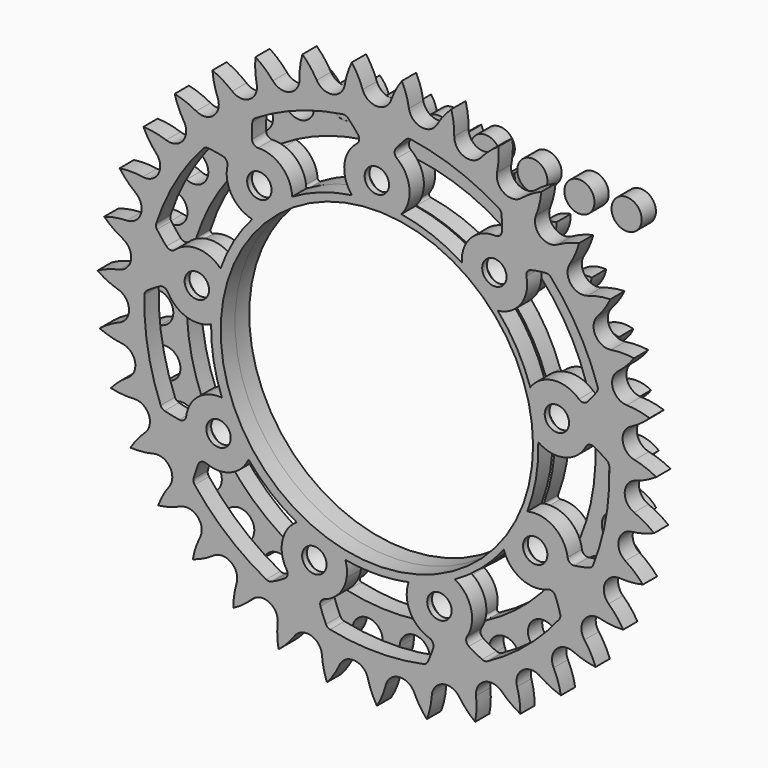
from build123d import *

# Parameters (mm, degrees)
F0_R           = 52.55
F1_DEPTH       = 6
F0_R_2         = 5.07
F2_D           = 8.2
F2_CSINK_D     = 16.2
F2_CSINK_ANGLE = 90
F3_R           = 52.55
F4_DEPTH       = 6
F5_D           = 8.2
F5_CSINK_D     = 16.2
F5_CSINK_ANGLE = 90
F6_D           = 8.2
F6_CSINK_D     = 16.2
F6_CSINK_ANGLE = 90


# Not quite as in the source:
# - a feature names something its author has since deleted; it is built from what else it names


with BuildPart() as f1:
    # F0 (on Front) → F1 (new body)
    with BuildSketch(Plane.XZ):
        with BuildLine():
            ThreePointArc((5.0539361628, 77.9443789243), (0, 73.378314), (-5.0539361628, 77.9443789243))
            ThreePointArc((-5.0539361628, 77.9443789243), (-6.1871728917, 81.776647272), (-8.6369474048, 84.9340371763))
            ThreePointArc((-8.6369474048, 84.9340371763), (-10.4009969746, 81.3481432448), (-10.739606334, 77.3662027789))
            ThreePointArc((-10.739606334, 77.3662027789), (-14.7709460148, 71.8762556016), (-20.6405699194, 75.3315030385))
            ThreePointArc((-20.6405699194, 75.3315030385), (-22.5220391728, 78.8572057516), (-25.5572445727, 81.456827715))
            ThreePointArc((-25.5572445727, 81.456827715), (-26.5633488026, 77.5892366752), (-26.0934680857, 73.6206452016))
            ThreePointArc((-26.0934680857, 73.6206452016), (-28.9371677642, 67.4315748538), (-35.3821763182, 69.6345465672))
            ThreePointArc((-35.3821763182, 69.6345465672), (-37.9348505239, 72.7093409623), (-41.4312251451, 74.6447661563))
            ThreePointArc((-41.4312251451, 74.6447661563), (-41.6381940096, 70.6538176397), (-40.3790601881, 66.8610497596))
            ThreePointArc((-40.3790601881, 66.8610497596), (-41.9186984654, 60.2262375086), (-48.6752322614, 61.0867435777))
            ThreePointArc((-48.6752322614, 61.0867435777), (-51.7946046375, 63.5847472111), (-55.609006492, 64.7767391007))
            ThreePointArc((-55.609006492, 64.7767391007), (-55.0083666616, 60.8258230086), (-53.0115288221, 57.3641550847))
            ThreePointArc((-53.0115288221, 57.3641550847), (-53.1840727262, 50.5552309235), (-59.9755184767, 50.0380421288))
            ThreePointArc((-59.9755184767, 50.0380421288), (-63.5338815515, 51.8569864381), (-67.5101485793, 52.2567447354))
            ThreePointArc((-67.5101485793, 52.2567447354), (-66.1264903192, 48.5076120368), (-63.4736992375, 45.5187651606))
            ThreePointArc((-63.4736992375, 45.5187651606), (-62.2720848007, 38.8144872445), (-68.8203999187, 36.9407773559))
            ThreePointArc((-68.8203999187, 36.9407773559), (-72.67207389, 38.0061945474), (-76.6474172517, 37.5973531007))
            ThreePointArc((-76.6474172517, 37.5973531007), (-74.5373876936, 34.2034937288), (-71.3372489483, 31.8098316426))
            ThreePointArc((-71.3372489483, 31.8098316426), (-68.8106704069, 25.4846738971), (-74.847766102, 22.3311528177))
            ThreePointArc((-74.847766102, 22.3311528177), (-78.8350629847, 22.5994245865), (-82.6467316562, 21.3987214126))
            ThreePointArc((-82.6467316562, 21.3987214126), (-79.8967156581, 18.4990803688), (-76.2802433053, 16.7985998796))
            ThreePointArc((-76.2802433053, 16.7985998796), (-72.5321390816, 11.1115150061), (-77.8108559469, 6.8072882593))
            ThreePointArc((-77.8108559469, 6.8072882593), (-81.7705353382, 6.2674315276), (-85.262479156, 4.3240235556))
            ThreePointArc((-85.262479156, 4.3240235556), (-81.9850626961, 2.0373124849), (-78.1003155389, 1.0996314638))
            ThreePointArc((-78.1003155389, 1.0996314638), (-73.2841334602, -3.7165506149), (-77.5883602069, -8.9952674802))
            ThreePointArc((-77.5883602069, -8.9952674802), (-81.3583123673, -10.3211509144), (-84.3875707413, -12.9277003338))
            ThreePointArc((-84.3875707413, -12.9277003338), (-80.7169316345, -14.5078632114), (-76.7229516779, -14.6443559933))
            ThreePointArc((-76.7229516779, -14.6443559933), (-71.0358668044, -18.392460217), (-74.1893878838, -24.4295559122))
            ThreePointArc((-74.1893878838, -24.4295559122), (-77.6152705288, -26.4871842253), (-80.0578252653, -29.6501626526))
            ThreePointArc((-80.0578252653, -29.6501626526), (-76.1442399079, -30.4590852833), (-72.2045411607, -29.7888017954))
            ThreePointArc((-72.2045411607, -29.7888017954), (-65.8793834152, -32.3153803368), (-67.7530933038, -38.8636954547))
            ThreePointArc((-67.7530933038, -38.8636954547), (-70.6946503955, -41.5688291019), (-72.4505030166, -45.1587438287))
            ThreePointArc((-72.4505030166, -45.1587438287), (-68.4541940529, -45.1633088249), (-64.7300682447, -43.7136905519))
            ThreePointArc((-64.7300682447, -43.7136905519), (-58.0257903286, -44.9153049887), (-58.5429791233, -51.7067507391))
            ThreePointArc((-58.5429791233, -51.7067507391), (-60.8797829688, -54.9486412309), (-61.8770486618, -58.8185207264))
            ThreePointArc((-61.8770486618, -58.8185207264), (-57.9616254504, -58.0185411967), (-54.6055387293, -55.8489356812))
            ThreePointArc((-54.6055387293, -55.8489356812), (-47.7966145682, -55.676391777), (-46.936108499, -62.432925573))
            ThreePointArc((-46.936108499, -62.432925573), (-48.5724900742, -66.0788495317), (-48.7703406645, -70.0702604748))
            ThreePointArc((-48.7703406645, -70.0702604748), (-45.0961010917, -68.4984876751), (-42.2454520424, -65.6977188216))
            ThreePointArc((-42.2454520424, -65.6977188216), (-35.6106397914, -64.1580805443), (-33.407668078, -70.6030890983))
            ThreePointArc((-33.407668078, -70.6030890983), (-34.276633729, -74.5037819688), (-33.6669691902, -78.4533155264))
            ThreePointArc((-33.6669691902, -78.4533155264), (-30.3843370557, -76.1740980198), (-28.1558315853, -72.8568296344))
            ThreePointArc((-28.1558315853, -72.8568296344), (-21.9667612376, -70.0131299558), (-18.5115138007, -75.8827538604))
            ThreePointArc((-18.5115138007, -75.8827538604), (-18.5774879716, -79.8785208183), (-17.1852680415, -83.6244826225))
            ThreePointArc((-17.1852680415, -83.6244826225), (-14.4286346907, -80.7311318415), (-12.9135080749, -77.0331732816))
            ThreePointArc((-12.9135080749, -77.0331732816), (-7.4235608976, -73.0018336008), (-2.8574959733, -78.0557697636))
            ThreePointArc((-2.8574959733, -78.0557697636), (-2.1177776738, -81.9830236401), (0, -85.3720535746))
            ThreePointArc((0, -85.3720535746), (2.1177776738, -81.9830236401), (2.8574959733, -78.0557697636))
            ThreePointArc((2.8574959733, -78.0557697636), (7.4235608976, -73.0018336008), (12.9135080749, -77.0331732816))
            ThreePointArc((12.9135080749, -77.0331732816), (14.4286346907, -80.7311318415), (17.1852680415, -83.6244826225))
            ThreePointArc((17.1852680415, -83.6244826225), (18.5774879716, -79.8785208183), (18.5115138007, -75.8827538604))
            ThreePointArc((18.5115138007, -75.8827538604), (21.9667612376, -70.0131299558), (28.1558315853, -72.8568296344))
            ThreePointArc((28.1558315853, -72.8568296344), (30.3843370557, -76.1740980198), (33.6669691902, -78.4533155264))
            ThreePointArc((33.6669691902, -78.4533155264), (34.276633729, -74.5037819688), (33.407668078, -70.6030890983))
            ThreePointArc((33.407668078, -70.6030890983), (35.6106397914, -64.1580805443), (42.2454520424, -65.6977188216))
            ThreePointArc((42.2454520424, -65.6977188216), (45.0961010917, -68.4984876751), (48.7703406645, -70.0702604748))
            ThreePointArc((48.7703406645, -70.0702604748), (48.5724900742, -66.0788495317), (46.936108499, -62.432925573))
            ThreePointArc((46.936108499, -62.432925573), (47.7966145682, -55.676391777), (54.6055387293, -55.8489356812))
            ThreePointArc((54.6055387293, -55.8489356812), (57.9616254504, -58.0185411967), (61.8770486618, -58.8185207264))
            ThreePointArc((61.8770486618, -58.8185207264), (60.8797829688, -54.9486412309), (58.5429791233, -51.7067507391))
            ThreePointArc((58.5429791233, -51.7067507391), (58.0257903286, -44.9153049887), (64.7300682447, -43.7136905519))
            ThreePointArc((64.7300682447, -43.7136905519), (68.4541940529, -45.1633088249), (72.4505030166, -45.1587438287))
            ThreePointArc((72.4505030166, -45.1587438287), (70.6946503955, -41.5688291019), (67.7530933038, -38.8636954547))
            ThreePointArc((67.7530933038, -38.8636954547), (65.8793834152, -32.3153803368), (72.2045411607, -29.7888017954))
            ThreePointArc((72.2045411607, -29.7888017954), (76.1442399079, -30.4590852833), (80.0578252653, -29.6501626526))
            ThreePointArc((80.0578252653, -29.6501626526), (77.6152705288, -26.4871842253), (74.1893878838, -24.4295559122))
            ThreePointArc((74.1893878838, -24.4295559122), (71.0358668044, -18.392460217), (76.7229516779, -14.6443559933))
            ThreePointArc((76.7229516779, -14.6443559933), (80.7169316345, -14.5078632114), (84.3875707413, -12.9277003338))
            ThreePointArc((84.3875707413, -12.9277003338), (81.3583123673, -10.3211509144), (77.5883602069, -8.9952674802))
            ThreePointArc((77.5883602069, -8.9952674802), (73.2841334602, -3.7165506149), (78.1003155389, 1.0996314638))
            ThreePointArc((78.1003155389, 1.0996314638), (81.9850626961, 2.0373124849), (85.262479156, 4.3240235556))
            ThreePointArc((85.262479156, 4.3240235556), (81.7705353382, 6.2674315276), (77.8108559469, 6.8072882593))
            ThreePointArc((77.8108559469, 6.8072882593), (72.5321390816, 11.1115150061), (76.2802433053, 16.7985998796))
            ThreePointArc((76.2802433053, 16.7985998796), (79.8967156581, 18.4990803688), (82.6467316562, 21.3987214126))
            ThreePointArc((82.6467316562, 21.3987214126), (78.8350629847, 22.5994245865), (74.847766102, 22.3311528177))
            ThreePointArc((74.847766102, 22.3311528177), (68.8106704069, 25.4846738971), (71.3372489483, 31.8098316426))
            ThreePointArc((71.3372489483, 31.8098316426), (74.5373876936, 34.2034937288), (76.6474172517, 37.5973531007))
            ThreePointArc((76.6474172517, 37.5973531007), (72.67207389, 38.0061945474), (68.8203999187, 36.9407773559))
            ThreePointArc((68.8203999187, 36.9407773559), (62.2720848007, 38.8144872445), (63.4736992375, 45.5187651606))
            ThreePointArc((63.4736992375, 45.5187651606), (66.1264903192, 48.5076120368), (67.5101485793, 52.2567447354))
            ThreePointArc((67.5101485793, 52.2567447354), (63.5338815515, 51.8569864381), (59.9755184767, 50.0380421288))
            ThreePointArc((59.9755184767, 50.0380421288), (53.1840727262, 50.5552309235), (53.0115288221, 57.3641550847))
            ThreePointArc((53.0115288221, 57.3641550847), (55.0083666616, 60.8258230086), (55.609006492, 64.7767391007))
            ThreePointArc((55.609006492, 64.7767391007), (51.7946046375, 63.5847472111), (48.6752322614, 61.0867435777))
            ThreePointArc((48.6752322614, 61.0867435777), (41.9186984654, 60.2262375086), (40.3790601881, 66.8610497596))
            ThreePointArc((40.3790601881, 66.8610497596), (41.6381940096, 70.6538176397), (41.4312251451, 74.6447661563))
            ThreePointArc((41.4312251451, 74.6447661563), (37.9348505239, 72.7093409623), (35.3821763182, 69.6345465672))
            ThreePointArc((35.3821763182, 69.6345465672), (28.9371677642, 67.4315748538), (26.0934680857, 73.6206452016))
            ThreePointArc((26.0934680857, 73.6206452016), (26.5633488026, 77.5892366752), (25.5572445727, 81.456827715))
            ThreePointArc((25.5572445727, 81.456827715), (22.5220391728, 78.8572057516), (20.6405699194, 75.3315030385))
            ThreePointArc((20.6405699194, 75.3315030385), (14.7709460148, 71.8762556016), (10.739606334, 77.3662027789))
            ThreePointArc((10.739606334, 77.3662027789), (10.4009969746, 81.3481432448), (8.6369474048, 84.9340371763))
            ThreePointArc((8.6369474048, 84.9340371763), (6.1871728917, 81.776647272), (5.0539361628, 77.9443789243))
        make_face()
        with BuildLine():
            ThreePointArc((-54.4759158417, -41.93959675), (-54.5447016016, -41.1315886082), (-53.8383054337, -40.7333260165))
            ThreePointArc((-53.8383054337, -40.7333260165), (-48.0309187527, -39.2735438367), (-44.0987264454, -34.7575093225))
            ThreePointArc((-44.0987264454, -34.7575093225), (-43.5114164609, -34.3147443915), (-42.8280957261, -34.5868593957))
            ThreePointArc((-42.8280957261, -34.5868593957), (-35.3854239296, -42.1707055316), (-26.6243883257, -48.1833871988))
            ThreePointArc((-26.6243883257, -48.1833871988), (-26.2377500975, -48.8090744024), (-26.5718029893, -49.4643470644))
            ThreePointArc((-26.5718029893, -49.4643470644), (-30.3364098723, -54.1210028385), (-30.7655709797, -60.093651223))
            ThreePointArc((-30.7655709797, -60.093651223), (-31.0351185634, -60.8584733913), (-31.8427958991, -60.9310417763))
            ThreePointArc((-31.8427958991, -60.9310417763), (-44.1916130719, -52.665515334), (-54.4759158417, -41.93959675))
        make_face(mode=Mode.SUBTRACT)
        with BuildLine():
            ThreePointArc((-68.6892257605, 2.8888486924), (-68.2225410875, 3.5520334735), (-67.4254119691, 3.4030576147))
            ThreePointArc((-67.4254119691, 3.4030576147), (-62.0383657751, 0.7883994384), (-56.1232806782, 1.7203180889))
            ThreePointArc((-56.1232806782, 1.7203180889), (-55.3887713165, 1.6819801228), (-55.0402294178, 1.0342978342))
            ThreePointArc((-55.0402294178, 1.0342978342), (-54.2136143761, -9.5593225694), (-51.3671490125, -19.7967890831))
            ThreePointArc((-51.3671490125, -19.7967890831), (-51.4731509283, -20.524619551), (-52.1502514379, -20.8118624726))
            ThreePointArc((-52.1502514379, -20.8118624726), (-58.0273482552, -21.9592250922), (-62.1952491153, -26.2586797555))
            ThreePointArc((-62.1952491153, -26.2586797555), (-62.8933527575, -26.6713056804), (-63.558715551, -26.2077313044))
            ThreePointArc((-63.558715551, -26.2077313044), (-67.7054803406, -11.938304031), (-68.6892257605, 2.8888486924))
        make_face(mode=Mode.SUBTRACT)
        with BuildLine():
            ThreePointArc((10.5762195558, -54.0244429456), (11.274585604, -54.2552208885), (11.4398873906, -54.9719139298))
            ThreePointArc((11.4398873906, -54.9719139298), (11.5492718416, -60.9589618687), (15.0596597386, -65.8101354168))
            ThreePointArc((15.0596597386, -65.8101354168), (15.3447925233, -66.5692850359), (14.7727218472, -67.1440406279))
            ThreePointArc((14.7727218472, -67.1440406279), (1.0883e-06, -68.7499467003), (-14.7727194682, -67.1440387664))
            ThreePointArc((-14.7727194682, -67.1440387664), (-15.3447900394, -66.5692832535), (-15.0596574397, -65.810133704))
            ThreePointArc((-15.0596574397, -65.810133704), (-11.5492710417, -60.9589594738), (-11.4398880061, -54.9719118352))
            ThreePointArc((-11.4398880061, -54.9719118352), (-11.2745862677, -54.2552186391), (-10.5762200628, -54.0244407242))
            ThreePointArc((-10.5762200628, -54.0244407242), (-3.612e-07, -55.0499467003), (10.5762195558, -54.0244429456))
        make_face(mode=Mode.SUBTRACT)
        with BuildLine():
            ThreePointArc((31.842796525, -60.9310388211), (31.0351193206, -60.8584704293), (30.7655716397, -60.0936484332))
            ThreePointArc((30.7655716397, -60.0936484332), (30.3364089456, -54.1210004897), (26.5718011715, -49.4643458555))
            ThreePointArc((26.5718011715, -49.4643458555), (26.2377481432, -48.8090731059), (26.6243865094, -48.183385823))
            ThreePointArc((26.6243865094, -48.183385823), (35.3854233761, -42.1707059959), (42.8280967655, -34.5868614233))
            ThreePointArc((42.8280967655, -34.5868614233), (43.5114173983, -34.3147465412), (44.0987273203, -34.7575113226))
            ThreePointArc((44.0987273203, -34.7575113226), (48.0309209049, -39.2735451572), (53.8383082957, -40.7333258508))
            ThreePointArc((53.8383082957, -40.7333258508), (54.5447046501, -41.1315883769), (54.4759188607, -41.9395966468))
            ThreePointArc((54.4759188607, -41.9395966468), (44.1916147393, -52.6655139349), (31.842796525, -60.9310388211))
        make_face(mode=Mode.SUBTRACT)
        with BuildLine():
            ThreePointArc((63.5587141308, -26.2077286383), (62.8933514335, -26.6713029247), (62.1952478277, -26.2586771941))
            ThreePointArc((62.1952478277, -26.2586771941), (58.0273460356, -21.9592238886), (52.1502492683, -20.8118627151))
            ThreePointArc((52.1502492683, -20.8118627151), (51.4731485978, -20.524619814), (51.3671467368, -19.7967891966))
            ThreePointArc((51.3671467368, -19.7967891966), (54.2136142506, -9.5593232809), (55.0402315174, 1.0342969491))
            ThreePointArc((55.0402315174, 1.0342969491), (55.3887734164, 1.6819790786), (56.1232826341, 1.7203171191))
            ThreePointArc((56.1232826341, 1.7203171191), (62.0383682726, 0.7883998102), (67.4254140551, 3.4030595812))
            ThreePointArc((67.4254140551, 3.4030595812), (68.2225432742, 3.5520356103), (68.6892280069, 2.888850712))
            ThreePointArc((68.6892280069, 2.888850712), (67.7054807186, -11.9383018874), (63.5587141308, -26.2077286383))
        make_face(mode=Mode.SUBTRACT)
        with BuildLine():
            ThreePointArc((-50.7620835502, 46.3655697256), (-49.9782953896, 46.5736196166), (-49.4634188942, 45.9471127671))
            ThreePointArc((-49.4634188942, 45.9471127671), (-47.0173719717, 40.4814418542), (-41.8871281409, 37.3931895473))
            ThreePointArc((-41.8871281409, 37.3931895473), (-41.3491044955, 36.8916874445), (-41.498428061, 36.1714956125))
            ThreePointArc((-41.498428061, 36.1714956125), (-47.6746521388, 27.524973663), (-52.074649794, 17.8529466615))
            ThreePointArc((-52.074649794, 17.8529466615), (-52.6236923793, 17.3635328941), (-53.3270176532, 17.5787238682))
            ThreePointArc((-53.3270176532, 17.5787238682), (-58.5666454874, 20.4775181244), (-64.5230789667, 19.8630198024))
            ThreePointArc((-64.5230789667, 19.8630198024), (-65.3230882145, 19.9956623769), (-65.5348058201, 20.7784679112))
            ThreePointArc((-65.5348058201, 20.7784679112), (-59.5392008954, 34.3749724076), (-50.7620835502, 46.3655697256))
        make_face(mode=Mode.SUBTRACT)
        with BuildLine():
            ThreePointArc((-9.0827982891, 68.1473253883), (-8.348649832, 67.8028915329), (-8.356942394, 66.9920032105))
            ThreePointArc((-8.356942394, 66.9920032105), (-9.9964272829, 61.2327677253), (-8.0515228228, 55.5693720375))
            ThreePointArc((-8.0515228228, 55.5693720375), (-7.9617321369, 54.8393642055), (-8.5390510107, 54.3836485923))
            ThreePointArc((-8.5390510107, 54.3836485923), (-18.8281903211, 51.7300288125), (-28.4158431917, 47.1490902497))
            ThreePointArc((-28.4158431917, 47.1490902497), (-29.1510233189, 47.1270953238), (-29.5514796447, 47.7440299453))
            ThreePointArc((-29.5514796447, 47.7440299453), (-31.7019584003, 53.3326030283), (-36.6598430755, 56.6905916418))
            ThreePointArc((-36.6598430755, 56.6905916418), (-37.1874247107, 57.3064377811), (-36.8464321078, 58.0421910643))
            ThreePointArc((-36.8464321078, 58.0421910643), (-23.5138676467, 64.6038172215), (-9.0827982891, 68.1473253883))
        make_face(mode=Mode.SUBTRACT)
        with Locations((5.4201e-06, 5.32997e-05)):
            Circle(F0_R, mode=Mode.SUBTRACT)
        with BuildLine():
            ThreePointArc((65.5348030184, 20.7784690407), (65.3230854289, 19.9956636369), (64.523076334, 19.8630209369))
            ThreePointArc((64.523076334, 19.8630209369), (58.5666430134, 20.4775176196), (53.327016147, 17.5787222879))
            ThreePointArc((53.327016147, 17.5787222879), (52.6236907632, 17.3635311946), (52.0746481238, 17.8529451117))
            ThreePointArc((52.0746481238, 17.8529451117), (47.6746525, 27.5249730373), (41.4984302383, 36.1714962841))
            ThreePointArc((41.4984302383, 36.1714962841), (41.3491067754, 36.8916879944), (41.8871302625, 37.3931900616))
            ThreePointArc((41.8871302625, 37.3931900616), (47.0173736459, 40.4814437444), (49.4634192281, 45.9471156144))
            ThreePointArc((49.4634192281, 45.9471156144), (49.9782956912, 46.5736226589), (50.7620839729, 46.3655727167))
            ThreePointArc((50.7620839729, 46.3655727167), (59.5391998071, 34.3749742927), (65.5348030184, 20.7784690407))
        make_face(mode=Mode.SUBTRACT)
        with BuildLine():
            ThreePointArc((36.8464292355, 58.0421901287), (37.1874217669, 57.3064369558), (36.6598403294, 56.6905908186))
            ThreePointArc((36.6598403294, 56.6905908186), (31.7019568296, 53.3326010513), (29.5514795067, 47.7440277666))
            ThreePointArc((29.5514795067, 47.7440277666), (29.1510231733, 47.1270929831), (28.4158429084, 47.1490879889))
            ThreePointArc((28.4158429084, 47.1490879889), (18.8281909999, 51.7300285654), (8.539052247, 54.3836505063))
            ThreePointArc((8.539052247, 54.3836505063), (7.96173353, 54.8393660922), (8.0515241176, 55.5693737953))
            ThreePointArc((8.0515241176, 55.5693737953), (9.9964273504, 61.2327702494), (8.3569408196, 66.9920056063))
            ThreePointArc((8.3569408196, 66.9920056063), (8.3486481074, 67.8028940573), (9.0827966903, 68.1473279513))
            ThreePointArc((9.0827966903, 68.1473279513), (23.5138656014, 64.6038179659), (36.8464292355, 58.0421901287))
        make_face(mode=Mode.SUBTRACT)
    extrude(amount=-F1_DEPTH)

    # F2 (through all)
    with Locations(Plane.XZ):
        with Locations((-60.5657293002, 10.6793721819), (-39.5314722561, 47.1117740818), (0, 61.5000532997), (39.5314722561, 47.1117740818), (60.5657293002, 10.6793721819), (53.2606084916, -30.7500266499), (21.0342570441, -57.7911462637), (-21.0342570441, -57.7911462637), (-53.2606084916, -30.7500266499)):
            CounterSinkHole(F2_D / 2, F2_CSINK_D / 2, counter_sink_angle=F2_CSINK_ANGLE)


with BuildPart() as f1b:
    # F0 (on Front) → F1, piece 2 (new body)
    with BuildSketch(Plane.XZ):
        with Locations((-15.7935424969, 76.8522677032)):
            Circle(F0_R_2)
    extrude(amount=-F1_DEPTH)


with BuildPart() as f1c:
    # F0 (on Front) → F1, piece 3 (new body)
    with BuildSketch(Plane.XZ):
        with Locations((0, 78.458314)):
            Circle(F0_R_2)
    extrude(amount=-F1_DEPTH)


with BuildPart() as f1d:
    # F0 (on Front) → F1, piece 4 (new body)
    with BuildSketch(Plane.XZ):
        with Locations((15.8799886703, 78.458314)):
            Circle(F0_R_2)
    extrude(amount=-F1_DEPTH)


with BuildPart() as f1e:
    # F0 (on Front) → F1, piece 5 (new body)
    with BuildSketch(Plane.XZ):
        with Locations((31.7430435847, 77.8425918352)):
            Circle(F0_R_2)
    extrude(amount=-F1_DEPTH)


with BuildPart() as f1f:
    # F0 (on Front) → F1, piece 6 (new body)
    with BuildSketch(Plane.XZ):
        with Locations((47.5038162957, 75.9416266721)):
            Circle(F0_R_2)
    extrude(amount=-F1_DEPTH)


with BuildPart() as f1g:
    # F0 (on Front) → F1, piece 7 (new body)
    with BuildSketch(Plane.XZ):
        with Locations((63.3414363061, 74.8528579142)):
            Circle(F0_R_2)
    extrude(amount=-F1_DEPTH)


with BuildPart() as f1h:
    # F0 (on Front) → F1, piece 8 (new body)
    with BuildSketch(Plane.XZ):
        with Locations((79.2164363061, 74.8528579142)):
            Circle(F0_R_2)
    extrude(amount=-F1_DEPTH)


with BuildPart() as f4:
    # F3 (on Front) → F4 (new body)
    with BuildSketch(Plane.XZ):
        with BuildLine():
            ThreePointArc((4.7900344729, 86.8582642793), (2.88e-07, 83.47), (-4.7900342811, 86.8582637362))
            ThreePointArc((-4.7900342811, 86.8582637362), (-6.3574974769, 90.4284112682), (-8.4356319096, 93.7275401761))
            ThreePointArc((-8.4356319096, 93.7275401761), (-9.8912869388, 90.1103646743), (-10.796085309, 86.3177099202))
            ThreePointArc((-10.796085309, 86.3177099202), (-14.9041437255, 82.1286028118), (-20.2221983199, 84.6071220571))
            ThreePointArc((-20.2221983199, 84.6071220571), (-22.4019461946, 87.8400144886), (-25.0357663654, 90.7150598063))
            ThreePointArc((-25.0357663654, 90.7150598063), (-25.8221567938, 86.8960965611), (-26.0352100261, 83.0028333418))
            ThreePointArc((-26.0352100261, 83.0028333418), (-29.3292562964, 78.1475247535), (-35.0044042658, 79.6366378602))
            ThreePointArc((-35.0044042658, 79.6366378602), (-37.7263779292, 82.4283673683), (-40.8312306906, 84.7869227739))
            ThreePointArc((-40.8312306906, 84.7869227739), (-40.9230812829, 80.8889164061), (-40.437541671, 77.0201774048))
            ThreePointArc((-40.437541671, 77.0201774048), (-42.8117024378, 71.6547209497), (-48.6615398569, 72.1065665972))
            ThreePointArc((-48.6615398569, 72.1065665972), (-51.8382528358, 74.3674046985), (-55.3143456654, 76.1336642805))
            ThreePointArc((-55.3143456654, 76.1336642805), (-54.708704268, 72.2818999222), (-53.5401774546, 68.5620295937))
            ThreePointArc((-53.5401774546, 68.5620295937), (-54.9181452373, 62.8588754568), (-60.7546535182, 62.2589309543))
            ThreePointArc((-60.7546535182, 62.2589309543), (-64.2840036436, 63.916212452), (-68.0196120578, 65.0334071742))
            ThreePointArc((-68.0196120578, 65.0334071742), (-66.7359444834, 61.351683701), (-64.9219878817, 57.9002417383))
            ThreePointArc((-64.9219878817, 57.9002417383), (-65.259473662, 52.0426939863), (-70.8950626263, 50.4102420436))
            ThreePointArc((-70.8950626263, 50.4102420436), (-74.6636136813, 51.4107005468), (-78.5386721518, 51.8429228516))
            ThreePointArc((-78.5386721518, 51.8429228516), (-76.6182365326, 48.4495738853), (-74.2171522003, 45.377492473))
            ThreePointArc((-74.2171522003, 45.377492473), (-73.5033089076, 39.5538175102), (-78.7568460889, 36.9413264761))
            ThreePointArc((-78.7568460889, 36.9413264761), (-82.6434737418, 37.2528064253), (-86.5334347011, 36.9861643321))
            ThreePointArc((-86.5334347011, 36.9861643321), (-84.037955418, 33.9902549005), (-81.1269161812, 31.3962732629))
            ThreePointArc((-81.1269161812, 31.3962732629), (-79.3846873262, 25.7936487944), (-84.0873197169, 22.2850862801))
            ThreePointArc((-84.0873197169, 22.2850862801), (-87.9671045569, 21.8975764534), (-91.7469414591, 20.9406400586))
            ThreePointArc((-91.7469414591, 20.9406400586), (-88.7566252695, 18.438461156), (-85.4291943245, 16.4059519972))
            ThreePointArc((-85.4291943245, 16.4059519972), (-82.7145765761, 11.2044509832), (-86.7151577019, 6.9125850749))
            ThreePointArc((-86.7151577019, 6.9125850749), (-90.4634002521, 5.838540357), (-94.011626029, 4.2220663837))
            ThreePointArc((-94.011626029, 4.2220663837), (-90.6225841557, 2.2940400987), (-86.9857078709, 0.8883299355))
            ThreePointArc((-86.9857078709, 0.8883299355), (-83.3859512771, -3.7448671016), (-86.5558991689, -8.6820923023))
            ThreePointArc((-86.5558991689, -8.6820923023), (-90.0521278295, -10.4081512304), (-93.2546995853, -12.6322079788))
            ThreePointArc((-93.2546995853, -12.6322079788), (-89.5758586227, -13.924113295), (-85.7464291942, -14.6578437813))
            ThreePointArc((-85.7464291942, -14.6578437813), (-81.3772328939, -18.5738220766), (-83.6146628182, -23.9977200893))
            ThreePointArc((-83.6146628182, -23.9977200893), (-86.7465059235, -26.3203162735), (-89.5004903667, -29.080472783))
            ThreePointArc((-89.5004903667, -29.080472783), (-85.6500912902, -29.6947342305), (-81.7511897308, -29.7329023385))
            ThreePointArc((-81.7511897308, -29.7329023385), (-76.7529832881, -32.8057991273), (-77.9859824061, -38.5420414072))
            ThreePointArc((-77.9859824061, -38.5420414072), (-80.6527799417, -41.3865246951), (-82.8696617465, -44.5940672645))
            ThreePointArc((-82.8696617465, -44.5940672645), (-78.9714595505, -44.510941975), (-75.1283997643, -43.8523209502))
            ThreePointArc((-75.1283997643, -43.8523209502), (-69.6618296468, -45.9833708014), (-69.8507683524, -51.8475898018))
            ThreePointArc((-69.8507683524, -51.8475898018), (-71.9668072513, -55.12253616), (-73.5753340124, -58.6743717319))
            ThreePointArc((-73.5753340124, -58.6743717319), (-69.754620123, -57.8965314206), (-66.0909212136, -56.5622898847))
            ThreePointArc((-66.0909212136, -56.5622898847), (-60.3316874827, -57.6829991028), (-59.4704931305, -63.4867139998))
            ThreePointArc((-59.4704931305, -63.4867139998), (-60.9677621614, -67.0868639578), (-61.9162345051, -70.8688336145))
            ThreePointArc((-61.9162345051, -70.8688336145), (-58.2958098104, -69.421278709), (-54.9292260753, -67.4543002828))
            ThreePointArc((-54.9292260753, -67.4543002828), (-49.0624352419, -67.5286483512), (-47.1787873269, -73.0853229729))
            ThreePointArc((-47.1787873269, -73.0853229729), (-48.0091630312, -76.8949647488), (-48.267096276, -80.7855128736))
            ThreePointArc((-48.267096276, -80.7855128736), (-44.9633242045, -78.7147689796), (-42.002060415, -76.1782739681))
            ThreePointArc((-42.002060415, -76.1782739681), (-36.2162759636, -75.2038712789), (-33.3707164797, -80.3349095307))
            ThreePointArc((-33.3707164797, -80.3349095307), (-33.507509899, -84.2315981033), (-33.0666138582, -88.1056792785))
            ThreePointArc((-33.0666138582, -88.1056792785), (-30.1856803628, -85.4783018086), (-27.7249139736, -82.4538152485))
            ThreePointArc((-27.7249139736, -82.4538152485), (-22.2060957771, -80.4619799057), (-18.4900833474, -85.0024659965))
            ThreePointArc((-18.4900833474, -85.0024659965), (-17.9288978287, -88.8609585888), (-16.8033432638, -92.5940566577))
            ThreePointArc((-16.8033432638, -92.5940566577), (-14.4378439173, -89.4944916856), (-12.5566659849, -86.0792230635))
            ThreePointArc((-12.5566659849, -86.0792230635), (-7.482193401, -83.133974294), (-3.0151637226, -86.9379732649))
            ThreePointArc((-3.0151637226, -86.9379732649), (-1.7740362302, -90.6342547502), (6.09e-07, -94.1063848693))
            ThreePointArc((6.09e-07, -94.1063848693), (1.7740367111, -90.6342549635), (3.0151635802, -86.937973823))
            ThreePointArc((3.0151635802, -86.937973823), (7.4821928273, -83.1339743456), (12.5566657452, -86.0792225397))
            ThreePointArc((12.5566657452, -86.0792225397), (14.4378443525, -89.4944913898), (16.8033444622, -92.5940564402))
            ThreePointArc((16.8033444622, -92.5940564402), (17.92889834, -88.8609587128), (18.490083307, -85.0024665711))
            ThreePointArc((18.490083307, -85.0024665711), (22.2060952218, -80.4619800589), (27.7249136442, -82.4538147759))
            ThreePointArc((27.7249136442, -82.4538147759), (30.1856807381, -85.4783014398), (33.0666149985, -88.1056788505))
            ThreePointArc((33.0666149985, -88.1056788505), (33.5075104243, -84.231598134), (33.3707165425, -80.3349101033))
            ThreePointArc((33.3707165425, -80.3349101033), (36.2162754447, -75.2038715288), (42.0020600065, -76.178273562))
            ThreePointArc((42.0020600065, -76.178273562), (44.963324508, -78.7147685498), (48.2670973215, -80.7855122489))
            ThreePointArc((48.2670973215, -80.7855122489), (48.0091635535, -76.8949646852), (47.1787874909, -73.085323525))
            ThreePointArc((47.1787874909, -73.085323525), (49.0624347759, -67.5286486898), (54.9292256009, -67.4542999561))
            ThreePointArc((54.9292256009, -67.4542999561), (58.2958100322, -69.4212782319), (61.9162354223, -70.8688328131))
            ThreePointArc((61.9162354223, -70.8688328131), (60.967762664, -67.086863802), (59.4704933905, -63.4867145138))
            ThreePointArc((59.4704933905, -63.4867145138), (60.3316870846, -57.6829995191), (66.0909206885, -56.562289648))
            ThreePointArc((66.0909206885, -56.562289648), (69.7546202561, -57.8965309116), (73.5753347718, -58.6743707797))
            ThreePointArc((73.5753347718, -58.6743707797), (71.966807718, -55.122535917), (69.8507687, -51.8475902611))
            ThreePointArc((69.8507687, -51.8475902611), (69.6618293295, -45.9833712822), (75.1283992054, -43.8523208111))
            ThreePointArc((75.1283992054, -43.8523208111), (78.9714595906, -44.5109414503), (82.8696623237, -44.5940661919))
            ThreePointArc((82.8696623237, -44.5940661919), (80.6527803575, -41.3865243726), (77.9859828301, -38.5420417971))
            ThreePointArc((77.9859828301, -38.5420417971), (76.7529830617, -32.805799657), (81.751189156, -29.7329023014))
            ThreePointArc((81.751189156, -29.7329023014), (85.650091236, -29.6947337071), (89.5004907431, -29.0804716246))
            ThreePointArc((89.5004907431, -29.0804716246), (86.746506275, -26.320315882), (83.614663305, -23.9977203972))
            ThreePointArc((83.614663305, -23.9977203972), (81.3772327657, -18.5738226381), (85.746428622, -14.6578438475))
            ThreePointArc((85.746428622, -14.6578438475), (89.5758584758, -13.9241127897), (93.2546997488, -12.6322067718))
            ThreePointArc((93.2546997488, -12.6322067718), (90.0521281055, -10.4081507824), (86.5558997029, -8.6820925183))
            ThreePointArc((86.5558997029, -8.6820925183), (83.3859512513, -3.7448676771), (86.9857073197, 0.8883297682))
            ThreePointArc((86.9857073197, 0.8883297682), (90.6225839211, 2.2940405696), (94.0116259744, 4.2220676004))
            ThreePointArc((94.0116259744, 4.2220676004), (90.4634004436, 5.8385408471), (86.7151582659, 6.9125849577))
            ThreePointArc((86.7151582659, 6.9125849577), (82.7145766534, 11.2044504124), (85.429193812, 16.4059517342))
            ThreePointArc((85.429193812, 16.4059517342), (88.7566249545, 18.4384615774), (91.7469411881, 20.9406412461))
            ThreePointArc((91.7469411881, 20.9406412461), (87.9671046579, 21.8975769698), (84.0873202927, 22.2850862655))
            ThreePointArc((84.0873202927, 22.2850862655), (79.3846875042, 25.7936482466), (81.1269157239, 31.3962729127))
            ThreePointArc((81.1269157239, 31.3962729127), (84.0379550328, 33.990255259), (86.5334342224, 36.9861654521))
            ThreePointArc((86.5334342224, 36.9861654521), (82.6434737489, 37.2528069514), (78.7568466581, 36.9413265645))
            ThreePointArc((78.7568466581, 36.9413265645), (73.5033091806, 39.553817003), (74.217151813, 45.3774920467))
            ThreePointArc((74.217151813, 45.3774920467), (76.6182360896, 48.4495741692), (78.5386714808, 51.8429238681))
            ThreePointArc((78.5386714808, 51.8429238681), (74.6636135943, 51.4107010658), (70.8950631705, 50.4102422323))
            ThreePointArc((70.8950631705, 50.4102422323), (65.2594740212, 52.042693536), (64.9219875767, 57.9002412497))
            ThreePointArc((64.9219875767, 57.9002412497), (66.7359439969, 61.3516839012), (68.019611216, 65.0334080545))
            ThreePointArc((68.019611216, 65.0334080545), (64.2840034654, 63.9162129471), (60.75465402, 62.2589312371))
            ThreePointArc((60.75465402, 62.2589312371), (54.9181456711, 62.8588750778), (53.5401772417, 68.5620290584))
            ThreePointArc((53.5401772417, 68.5620290584), (54.7087037535, 72.2819000323), (55.31434468, 76.1336649964))
            ThreePointArc((55.31434468, 76.1336649964), (51.8382525721, 74.3674051538), (48.6615403002, 72.1065669651))
            ThreePointArc((48.6615403002, 72.1065669651), (42.8117029323, 71.6547206542), (40.4375415571, 77.0201768402))
            ThreePointArc((40.4375415571, 77.0201768402), (40.923080757, 80.8889164226), (40.8312295932, 84.7869233023))
            ThreePointArc((40.8312295932, 84.7869233023), (37.7263775885, 82.4283677692), (35.0044046362, 79.6366383013))
            ThreePointArc((35.0044046362, 79.6366383013), (29.3292568357, 78.1475245511), (26.0352100148, 83.0028327659))
            ThreePointArc((26.0352100148, 83.0028327659), (25.8221562734, 86.8960964834), (25.0357651913, 90.7150601304))
            ThreePointArc((25.0357651913, 90.7150601304), (22.4019457877, 87.8400148222), (20.2221986056, 84.6071225573))
            ThreePointArc((20.2221986056, 84.6071225573), (14.9041442922, 82.1286027089), (10.7960854008, 86.3177093516))
            ThreePointArc((10.7960854008, 86.3177093516), (9.8912864406, 90.1103645049), (8.4356306965, 93.7275402852))
            ThreePointArc((8.4356306965, 93.7275402852), (6.357497017, 90.4284115238), (4.7900344729, 86.8582642793))
        make_face()
        with BuildLine():
            ThreePointArc((-43.1839486307, -35.1455521405), (-35.7124281126, -42.6096343793), (-26.953056521, -48.5095963996))
            ThreePointArc((-26.953056521, -48.5095963996), (-31.7729548393, -55.3833001523), (-30.3400953245, -63.6553093815))
            ThreePointArc((-30.3400953245, -63.6553093815), (-30.0816101185, -65.1683120375), (-30.9715269517, -66.4189277532))
            ThreePointArc((-30.9715269517, -66.4189277532), (-33.1586851366, -67.6957261094), (-35.4187096835, -68.8386014375))
            ThreePointArc((-35.4187096835, -68.8386014375), (-36.322967339, -69.0266906549), (-37.2153152887, -68.7884164475))
            ThreePointArc((-37.2153152887, -68.7884164475), (-50.2888955627, -59.9202001432), (-61.2925854075, -48.5851848632))
            ThreePointArc((-61.2925854075, -48.5851848632), (-61.6821941451, -47.7477695928), (-61.6539850431, -46.8245883808))
            ThreePointArc((-61.6539850431, -46.8245883808), (-60.9209219757, -44.4004417863), (-60.0433175155, -42.0247990135))
            ThreePointArc((-60.0433175155, -42.0247990135), (-58.966233899, -40.9312348765), (-57.4313316681, -40.9230629575))
            ThreePointArc((-57.4313316681, -40.9230629575), (-49.1307256625, -40.9365870994), (-43.1839486307, -35.1455521405))
        make_face(mode=Mode.SUBTRACT)
        with BuildLine():
            ThreePointArc((-55.7632219307, 0.7992935259), (-54.9344258128, -9.6708962063), (-52.1322256225, -19.7931217585))
            ThreePointArc((-52.1322256225, -19.7931217585), (-60.0623218414, -22.0881118589), (-64.1625743097, -29.2533986848))
            ThreePointArc((-64.1625743097, -29.2533986848), (-64.9371025146, -30.5785770495), (-66.4226986461, -30.964576755))
            ThreePointArc((-66.4226986461, -30.964576755), (-68.9188691833, -30.5367828591), (-71.3847745291, -29.959560377))
            ThreePointArc((-71.3847745291, -29.959560377), (-72.1983774997, -29.5223994599), (-72.7287959796, -28.7662806218))
            ThreePointArc((-72.7287959796, -28.7662806218), (-77.0433599398, -13.5692973872), (-78.1866680217, 2.1868635739))
            ThreePointArc((-78.1866680217, 2.1868635739), (-77.9468454701, 3.0787965575), (-77.3318265996, 3.7678619337))
            ThreePointArc((-77.3318265996, 3.7678619337), (-75.2120563154, 5.1536621049), (-73.0127385561, 6.4093967766))
            ThreePointArc((-73.0127385561, 6.4093967766), (-71.4847151592, 6.5547795036), (-70.3036590262, 5.5744234207))
            ThreePointArc((-70.3036590262, 5.5744234207), (-64.0000085876, 0.2436248653), (-55.7632219307, 0.7992935259))
        make_face(mode=Mode.SUBTRACT)
        with BuildLine():
            ThreePointArc((5.3105962893, -54.8301701183), (8.0278304795, -54.4619576085), (10.7233586554, -53.9588970258))
            ThreePointArc((10.7233586554, -53.9588970258), (10.1067282391, -56.5303374291), (10.1215940367, -59.1746365472))
            ThreePointArc((10.1215940367, -59.1746365472), (12.5760906517, -64.823857347), (17.6825487, -68.2680314829))
            ThreePointArc((17.6825487, -68.2680314829), (18.8530992164, -69.2609076722), (18.975263658, -70.7909624058))
            ThreePointArc((18.975263658, -70.7909624058), (18.1205134477, -73.1749248732), (17.1238603025, -75.5031339438))
            ThreePointArc((17.1238603025, -75.5031339438), (16.5520601688, -76.2284642604), (15.7153222724, -76.6195258335))
            ThreePointArc((15.7153222724, -76.6195258335), (-8.086e-07, -78.2296134277), (-15.7153236456, -76.6195234528))
            ThreePointArc((-15.7153236456, -76.6195234528), (-16.5520614141, -76.2284618075), (-17.1238614327, -75.5031315088))
            ThreePointArc((-17.1238614327, -75.5031315088), (-18.1205139385, -73.1749236239), (-18.975263658, -70.7909624058))
            ThreePointArc((-18.975263658, -70.7909624058), (-18.8530992164, -69.2609076722), (-17.6825487, -68.2680314829))
            ThreePointArc((-17.6825487, -68.2680314829), (-12.6544540896, -64.917049305), (-10.1548949033, -59.4158657193))
            ThreePointArc((-10.1548949033, -59.4158657193), (-10.0777992921, -56.8131222566), (-10.6146461638, -54.2651794192))
            ThreePointArc((-10.6146461638, -54.2651794192), (-7.9582274938, -54.6837375456), (-5.2845379002, -54.9720689737))
            ThreePointArc((-5.2845379002, -54.9720689737), (0.0164512429, -55.15663296), (5.3105962893, -54.8301701183))
        make_face(mode=Mode.SUBTRACT)
        with BuildLine():
            ThreePointArc((26.2470836806, -48.1036313649), (35.1971419476, -41.8297543894), (42.7312849898, -33.911309851))
            ThreePointArc((42.7312849898, -33.911309851), (48.5277853029, -40.6791830862), (57.4350289125, -40.933221053))
            ThreePointArc((57.4350289125, -40.933221053), (58.9699311434, -40.941392972), (60.0470147599, -42.0349571089))
            ThreePointArc((60.0470147599, -42.0349571089), (60.9246196471, -44.4106011543), (61.6576829868, -46.8347490681))
            ThreePointArc((61.6576829868, -46.8347490681), (61.6858920123, -47.7579303678), (61.2962831302, -48.5953456651))
            ThreePointArc((61.2962831302, -48.5953456651), (50.2925915683, -59.9303592782), (37.2190099508, -68.7985736019))
            ThreePointArc((37.2190099508, -68.7985736019), (36.3266620527, -69.0368476717), (35.4224044969, -68.8487583942))
            ThreePointArc((35.4224044969, -68.8487583942), (33.1623812019, -67.7058835634), (30.9752241961, -66.4290858487))
            ThreePointArc((30.9752241961, -66.4290858487), (30.0853073629, -65.1784701329), (30.3437925689, -63.665467477))
            ThreePointArc((30.3437925689, -63.665467477), (31.6793741686, -54.993716182), (26.2470836806, -48.1036313649))
        make_face(mode=Mode.SUBTRACT)
        with BuildLine():
            ThreePointArc((50.5774174633, -20.0865459388), (53.5386445982, -9.4077902952), (54.3011244865, 1.6476749894))
            ThreePointArc((54.3011244865, 1.6476749894), (63.1905965579, -0.0070325802), (70.316718022, 5.5588603155))
            ThreePointArc((70.316718022, 5.5588603155), (71.497774155, 6.5392163984), (73.0257975519, 6.3938336714))
            ThreePointArc((73.0257975519, 6.3938336714), (75.2251164563, 5.1380982994), (77.3448877972, 3.7522972926))
            ThreePointArc((77.3448877972, 3.7522972926), (77.9599066654, 3.0632318001), (78.1997291235, 2.1712987029))
            ThreePointArc((78.1997291235, 2.1712987029), (77.0564186548, -13.5848620849), (72.7418523925, -28.7818446659))
            ThreePointArc((72.7418523925, -28.7818446659), (72.2114338635, -29.5379633654), (71.3978309306, -29.9751241724))
            ThreePointArc((71.3978309306, -29.9751241724), (68.9319268636, -30.5523462307), (66.435757642, -30.9801398602))
            ThreePointArc((66.435757642, -30.9801398602), (64.9501615104, -30.5941401547), (64.1756333055, -29.26896179))
            ThreePointArc((64.1756333055, -29.26896179), (59.4317198984, -21.6342216337), (50.5774174633, -20.0865459388))
        make_face(mode=Mode.SUBTRACT)
        with BuildLine():
            ThreePointArc((-41.9237828898, 36.3961454713), (-48.1353967691, 27.8590318867), (-52.6030286824, 18.2931173758))
            ThreePointArc((-52.6030286824, 18.2931173758), (-60.169549533, 21.6925616645), (-67.9589744434, 18.8406642577))
            ThreePointArc((-67.9589744434, 18.8406642577), (-69.4041057043, 18.3233758687), (-70.7902541936, 18.9826057256))
            ThreePointArc((-70.7902541936, 18.9826057256), (-72.4274511469, 20.9148223553), (-73.9454127747, 22.9420538331))
            ThreePointArc((-73.9454127747, 22.9420538331), (-74.2876671883, 23.7999124331), (-74.2079674968, 24.7200794942))
            ThreePointArc((-74.2079674968, 24.7200794942), (-67.7446827152, 39.1349923081), (-58.492642476, 51.9398161262))
            ThreePointArc((-58.492642476, 51.9398161262), (-57.7356042725, 52.4689214673), (-56.8215497983, 52.6014496601))
            ThreePointArc((-56.8215497983, 52.6014496601), (-54.3069363719, 52.3004721064), (-51.8149905356, 51.8487264682))
            ThreePointArc((-51.8149905356, 51.8487264682), (-50.5510064879, 50.9779015916), (-50.2764257434, 49.4677370133))
            ThreePointArc((-50.2764257434, 49.4677370133), (-48.7965136259, 41.208957176), (-41.9237828898, 36.3961454713))
        make_face(mode=Mode.SUBTRACT)
        with BuildLine():
            ThreePointArc((-8.3756621814, 54.4036114494), (-18.7913905159, 51.8879954331), (-28.5224823295, 47.4022878193))
            ThreePointArc((-28.5224823295, 47.4022878193), (-31.9940036864, 55.1549124039), (-39.9529179108, 58.1231328891))
            ThreePointArc((-39.9529179108, 58.1231328891), (-41.3924592498, 58.6557794621), (-42.0305658134, 60.0517779049))
            ThreePointArc((-42.0305658134, 60.0517779049), (-42.042726533, 62.5843116332), (-41.9024733269, 65.112987968))
            ThreePointArc((-41.9024733269, 65.112987968), (-41.6132345396, 65.9901426779), (-40.9607090481, 66.6438015676))
            ThreePointArc((-40.9607090481, 66.6438015676), (-26.7438183054, 73.5317460512), (-11.4255621982, 77.3937133522))
            ThreePointArc((-11.4255621982, 77.3937133522), (-10.5055349317, 77.3124167813), (-9.7201411008, 76.8263963763))
            ThreePointArc((-9.7201411008, 76.8263963763), (-7.9873001012, 74.9794718401), (-6.3687353397, 73.0316226967))
            ThreePointArc((-6.3687353397, 73.0316226967), (-5.9602228247, 71.5520588543), (-6.7205968506, 70.2187085706))
            ThreePointArc((-6.7205968506, 70.2187085706), (-10.9279707126, 62.664863686), (-8.3756621814, 54.4036114494))
        make_face(mode=Mode.SUBTRACT)
        Circle(F3_R, mode=Mode.SUBTRACT)
        with BuildLine():
            ThreePointArc((51.5945179846, 17.0236105583), (47.103970691, 27.1519193671), (40.6763277267, 36.175946198))
            ThreePointArc((40.6763277267, 36.175946198), (48.4576080697, 40.6628302451), (50.3001305301, 49.4540510483))
            ThreePointArc((50.3001305301, 49.4540510483), (50.5747112747, 50.9642156266), (51.8386953223, 51.8350405032))
            ThreePointArc((51.8386953223, 51.8350405032), (54.330642486, 52.2867863409), (56.845257259, 52.5877639337))
            ThreePointArc((56.845257259, 52.5877639337), (57.7593118062, 52.4552356504), (58.5163500111, 51.9261301623))
            ThreePointArc((58.5163500111, 51.9261301623), (67.7683883105, 39.1213049426), (74.2316709084, 24.7063911497))
            ThreePointArc((74.2316709084, 24.7063911497), (74.3113704733, 23.7862241632), (73.9691160178, 22.9283656718))
            ThreePointArc((73.9691160178, 22.9283656718), (72.4511550971, 20.9011353406), (70.8139589803, 18.9689197606))
            ThreePointArc((70.8139589803, 18.9689197606), (69.427810491, 18.3096899037), (67.9826792301, 18.8269782926))
            ThreePointArc((67.9826792301, 18.8269782926), (59.3820452195, 21.6198611782), (51.5945179846, 17.0236105583))
        make_face(mode=Mode.SUBTRACT)
        with BuildLine():
            ThreePointArc((28.567616184, 46.5005924693), (18.7869440373, 51.3661156578), (8.2380992961, 54.2045550471))
            ThreePointArc((8.2380992961, 54.2045550471), (10.9712295114, 62.5318222753), (6.7512501839, 70.2133035609))
            ThreePointArc((6.7512501839, 70.2133035609), (5.990876158, 71.5466538446), (6.399388673, 73.026217687))
            ThreePointArc((6.399388673, 73.026217687), (8.017954323, 74.9740678365), (9.750796329, 76.8209932682))
            ThreePointArc((9.750796329, 76.8209932682), (10.5361902741, 77.3070136507), (11.4562176361, 77.3883101099))
            ThreePointArc((11.4562176361, 77.3883101099), (26.7744731583, 73.5263404884), (40.9913628576, 66.6383938511))
            ThreePointArc((40.9913628576, 66.6383938511), (41.6438882041, 65.9847349372), (41.9331268895, 65.1075802836))
            ThreePointArc((41.9331268895, 65.1075802836), (42.0733799002, 62.5789052816), (42.0612191467, 60.0463728951))
            ThreePointArc((42.0612191467, 60.0463728951), (41.4231125831, 58.6503744524), (39.983571244, 58.1177278794))
            ThreePointArc((39.983571244, 58.1177278794), (31.7039937462, 54.8362263251), (28.567616184, 46.5005924693))
        make_face(mode=Mode.SUBTRACT)
    extrude(amount=F4_DEPTH)

    # F5 (through all)
    with Locations(Plane(origin=(0, 0, 0), x_dir=(1, 0, 0), z_dir=(0, 1, 0))):
        with Locations((0, -61.5), (39.5314379957, -47.1117332518), (60.5656768103, -10.6793629265), (53.2605623327, 30.75), (21.0342388145, 57.7910961783), (-21.0342388145, 57.7910961783), (-53.2605623327, 30.75)):
            CounterSinkHole(F5_D / 2, F5_CSINK_D / 2, counter_sink_angle=F5_CSINK_ANGLE)

    # F6 (through all)
    with Locations(Plane(origin=(0, 0, 0), x_dir=(1, 0, 0), z_dir=(0, 1, 0))):
        with Locations((-39.5313891572, -47.1115990699), (-60.5658174329, -10.6793381307)):
            CounterSinkHole(F6_D / 2, F6_CSINK_D / 2, counter_sink_angle=F6_CSINK_ANGLE)


solid = Compound([f1.part, f1b.part, f1c.part, f1d.part, f1e.part, f1f.part, f1g.part, f1h.part, f4.part])
